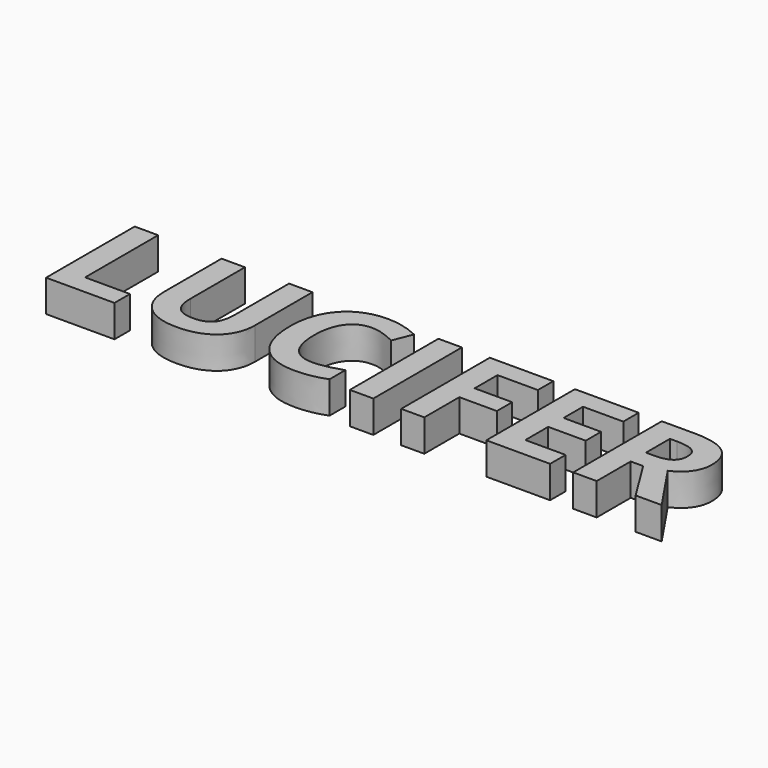
from build123d import *

# Parameters (mm, degrees)
F0_TEXT_SIZE = 122.9032304966
F1_DEPTH     = 25.4


# Not quite as in the source:
# - Text() gives the source's letters only with a copy of the font that has no kerning and outlines rounded to 1/6400 em; it was checked with that copy


with BuildPart() as f1:
    # F0 (on Top) → F1 (new body)
    with BuildSketch(Plane.XY):
        with Locations((-87.3841941357, -48.854034394)):
            Text('LUCIFER', F0_TEXT_SIZE, font='Open Sans', font_style=FontStyle.BOLD, text_align=(TextAlign.LEFT, TextAlign.BOTTOM))
    extrude(amount=F1_DEPTH)


solid = f1.part
